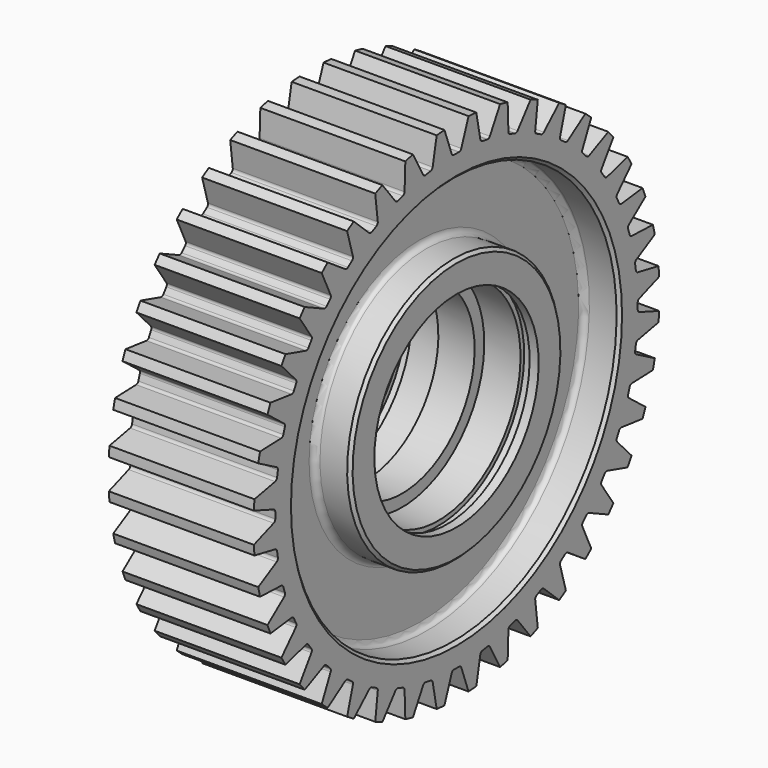
from build123d import *

# Parameters (mm, degrees)
F3_DEPTH        = 37.5
F3_COPIES_COUNT = 40
F5_SIZE2        = 1
F5_SIZE         = 1


# Not quite as in the source:
# - a feature of the source that left no trace in its solid (it failed there, or was rolled back) is left out
# - a pattern or mirror of a feature is missing from the dataset's text; its kind, count and spacing are read off the source's solid


with BuildPart() as f1:
    # F0 (on Front) → F1 (revolve)
    with BuildSketch(Plane.XZ):
        with BuildLine():
            Line((24, 84), (0, 84))
            Line((0, 84), (-24, 84))
            Line((-24, 84), (-24, 67.5))
            Line((-24, 67.5), (-14, 67.5))
            ThreePointArc((-14, 67.5), (-12.5857864376, 66.9142135624), (-12, 65.5))
            Line((-12, 65.5), (-12, 46))
            ThreePointArc((-12, 46), (-12.5857864376, 44.5857864376), (-14, 44))
            Line((-14, 44), (-24, 44))
            Line((-24, 44), (-24, 34))
            Line((-24, 34), (-21, 34))
            Line((-21, 34), (-21, 35.5))
            Line((-21, 35.5), (-18, 35.5))
            Line((-18, 35.5), (-18, 34))
            Line((-18, 34), (-6, 34))
            Line((-6, 34), (-6, 30))
            Line((-6, 30), (0, 30))
            Line((0, 30), (6, 30))
            Line((6, 30), (6, 34))
            Line((6, 34), (18, 34))
            Line((18, 34), (18, 35.5))
            Line((18, 35.5), (21, 35.5))
            Line((21, 35.5), (21, 34))
            Line((21, 34), (24, 34))
            Line((24, 34), (24, 44))
            Line((24, 44), (14, 44))
            ThreePointArc((14, 44), (12.5857864376, 44.5857864376), (12, 46))
            Line((12, 46), (12, 65.5))
            ThreePointArc((12, 65.5), (12.5857864376, 66.9142135624), (14, 67.5))
            Line((14, 67.5), (24, 67.5))
            Line((24, 67.5), (24, 84))
        make_face()
    revolve(axis=Axis((-13.5004352778, 0, 0), (-1, 0, 0)))

    # F2 (on Right) → F3 (cut, symmetric)
    with BuildSketch(Plane.YZ):
        with BuildLine():
            ThreePointArc((-1.0390922076, 74.9928015704), (0, 75), (1.0390922076, 74.9928015704))
            ThreePointArc((1.0390922076, 74.9928015704), (1.6208348109, 75.169599782), (1.9926393912, 75.6506854481))
            Line((1.9926393912, 75.6506854481), (4.9778115587, 83.8523785714))
            ThreePointArc((4.9778115587, 83.8523785714), (0, 84), (-4.9778115587, 83.8523785714))
            Line((-4.9778115587, 83.8523785714), (-1.9926393912, 75.6506854481))
            ThreePointArc((-1.9926393912, 75.6506854481), (-1.6208348109, 75.169599782), (-1.0390922076, 74.9928015704))
        make_face()
    f3 = extrude(amount=F3_DEPTH, both=True, mode=Mode.SUBTRACT)

    # F3_copies: F3 ×40 about axis
    f3_copies_axis = Axis((0, 0, 0), (1, 0, 0))
    for i in range(1, F3_COPIES_COUNT):
        add(f3.rotate(f3_copies_axis, i * 360 / F3_COPIES_COUNT), mode=Mode.SUBTRACT)

    # F5
    f5_edges = [f1.edges().sort_by_distance(p)[0] for p in [
        (24, 0, -67.5),
        (24, 0, -44),
        (-24, 0, -44),
        (-24, 0, -67.5),
    ]]
    chamfer(f5_edges, length=F5_SIZE, length2=F5_SIZE2)


solid = f1.part
